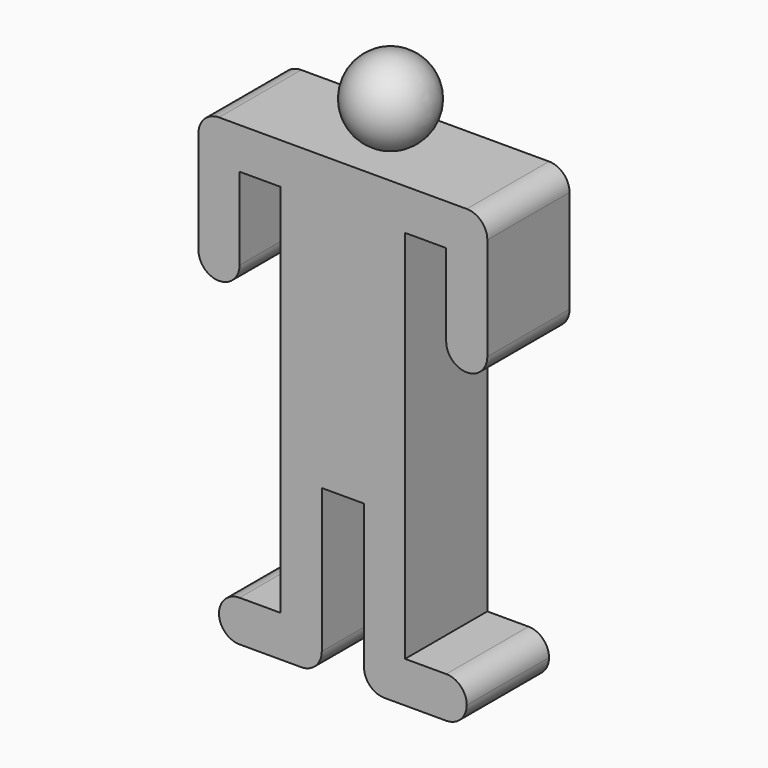
from build123d import *

# Parameters (mm, degrees)
F0_W          = 30.2604204044
F0_H          = 71.2152794003
F1_DEPTH      = 12.5
F1_DEPTH_BACK = 12.5
F4_W          = 15
F4_H          = 10
F4_W_2        = 10
F4_H_2        = 25
F5_DEPTH      = 12.5
F5_DEPTH_BACK = 12.5
F6_R          = 4.99999


# Not quite as in the source:
# - a fillet or chamfer is up to 0.001 mm smaller than in the source, because OpenCascade refuses the exact size


with BuildPart() as f1:
    # F0 (on Front) → F1 (new body, two sides)
    with BuildSketch(Plane.XZ) as f1_sk:
        with Locations((-1.579860691, 6.5017342567)):
            Rectangle(F0_W, F0_H)
    extrude(amount=F1_DEPTH)
    extrude(f1_sk.sketch, amount=-F1_DEPTH_BACK)

    # F4 (on Front) → F5 (join, two sides)
    with BuildSketch(Plane.XZ) as f5_sk:
        Polygon((13.5503495112, -29.1059054434), (3.5503495112, -29.1059054434), (3.5503495112, -69.1059054434), (13.5503495112, -69.1059054434), (13.5503495112, -59.1059054434), align=None)
        with Locations((21.0503495112, -64.1059054434)):
            Rectangle(F4_W, F4_H)
        Polygon((-6.7100708932, -69.1059054434), (-6.7100708932, -29.1059054434), (-16.7100708932, -29.1059054434), (-16.7100708932, -59.1059054434), (-16.7100708932, -69.1059054434), align=None)
        with Locations((-24.2100708932, -64.1059054434)):
            Rectangle(F4_W, F4_H)
        Polygon((-16.7100708932, 32.1093739569), (-16.7100708932, 42.1093739569), (-36.7100708932, 42.1093739569), (-36.7100708932, 32.1093739569), (-26.7100708932, 32.1093739569), align=None)
        with Locations((-31.7100708932, 19.6093739569)):
            Rectangle(F4_W_2, F4_H_2)
        Polygon((33.5503495112, 42.1093739569), (13.5503495112, 42.1093739569), (13.5503495112, 32.1093739569), (23.5503495112, 32.1093739569), (33.5503495112, 32.1093739569), align=None)
        with Locations((28.5503495112, 19.6093739569)):
            Rectangle(F4_W_2, F4_H_2)
    extrude(amount=F5_DEPTH)
    extrude(f5_sk.sketch, amount=-F5_DEPTH_BACK)

    # F6 (radius 5 in the source; OpenCascade refuses exactly that, so slightly less here)
    f6_edges = [f1.edges().sort_by_distance(p)[0] for p in [
        (-36.710071, 0, 42.109374),
        (33.55035, 0, 42.109374),
        (-6.710071, 0, -69.105905),
        (3.55035, 0, -69.105905),
        (-36.710071, 0, 7.109374),
        (23.55035, 0, 7.109374),
        (-31.710071, 0, -69.105905),
        (-31.710071, 0, -59.105905),
        (-26.710071, 0, 7.109374),
        (33.55035, 0, 7.109374),
        (28.55035, 0, -59.105905),
        (28.55035, 0, -69.105905),
    ]]
    fillet(f6_edges, radius=F6_R)


with BuildPart() as f3:
    # F2 (on Front) → F3 (revolve)
    with BuildSketch(Plane.XZ):
        with BuildLine():
            ThreePointArc((0, 41.3558275998), (10, 51.3558275998), (0, 61.3558275998))
            Line((0, 61.3558275998), (0, 41.3558275998))
        make_face()
    revolve(axis=Axis((0, 0, 51.3558275998), (0, 0, -1)))


solid = Compound([f1.part, f3.part])
